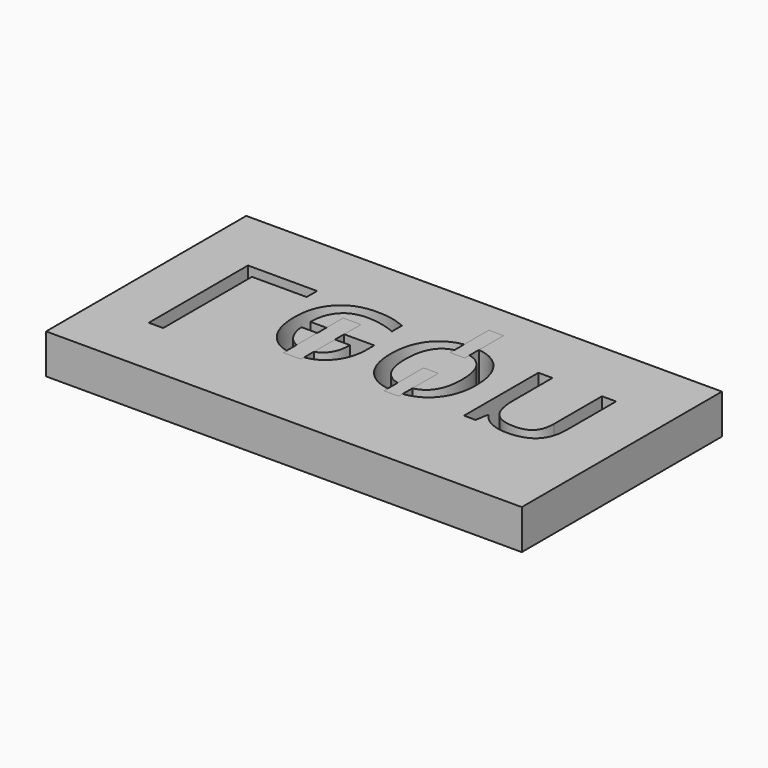
from build123d import *

# Parameters (mm, degrees)
F0_W         = 76.2
F0_H         = 40.0792241179
F1_DEPTH     = 6.35
F2_TEXT_SIZE = 27.8222769905
F3_DEPTH     = 48.006
F5_DEPTH     = 6.35
F4_W         = 2.8403475881
F4_H         = 3.3596433377


# Not quite as in the source:
# - Text() gives the source's letters only with a copy of the font that has no kerning and outlines rounded to 1/6400 em; it was checked with that copy


with BuildPart() as f1:
    # F0 (on Top) → F1 (new body)
    with BuildSketch(Plane.XY):
        Rectangle(F0_W, F0_H)
    extrude(amount=F1_DEPTH)

    # F2 (on face) → F3 (cut)
    with BuildSketch(Plane(origin=(0, 0, 0), x_dir=(1, 0, 0), z_dir=(0, 0, -1))):
        with Locations((-32.2671057508, -9.6827361845)):
            Text('Leon', F2_TEXT_SIZE, font='Open Sans', text_align=(TextAlign.LEFT, TextAlign.BOTTOM))
    extrude(amount=-F3_DEPTH, mode=Mode.SUBTRACT)


with BuildPart() as f5:
    # F4 (on face) → F5 (new body)
    with BuildSketch(Plane.XY.offset(6.35)):
        with BuildLine():
            Line((7.3115319722, 1.7436897615), (6.127636496, 1.7436897615))
            Line((6.127636496, 1.7436897615), (4.9437410198, 1.7436897615))
            Line((4.9437410198, 1.7436897615), (4.9437410198, -5.3931702091))
            add(Edge.make_bspline(
                [(4.9437410198, -5.3931702091), (5.1212427745, -5.4185774064), (5.2994799287, -5.4393437319), (5.4782769731, -5.4556621191), (5.6574797199, -5.4677304419), (5.8369560739, -5.475745273), (6.016596569, -5.4798974439), (6.2400864171, -5.4804843563), (6.2838595809, -5.4803749221), (6.3276294886, -5.4800287031), (6.3713925881, -5.4794371058), (6.4151464477, -5.4785953434), (6.4588897564, -5.4775024361), (6.6186138738, -5.4726038897), (6.7345245325, -5.4672766583), (6.8503204098, -5.4601261923), (6.965963384, -5.4510985496), (7.0814111862, -5.440139936), (7.1966174851, -5.42719747), (7.3115319723, -5.4122199485)],
                knots=[0.7306547471, 0.7306547471, 0.7306547471, 0.7306547471, 0.7306547471, 0.7306547471, 0.7306547471, 0.7306547471, 0.7570691699, 0.7570691699, 0.7570691699, 0.7570691699, 0.7570691699, 0.7570691699, 0.763502609, 0.763502609, 0.763502609, 0.763502609, 0.763502609, 0.763502609, 0.7805659698, 0.7805659698, 0.7805659698, 0.7805659698, 0.7805659698, 0.7805659698, 0.7805659698, 0.7805659698], degree=7))
            Line((7.3115319722, -5.4122199485), (7.3115319722, 1.7436897615))
        make_face()
        with BuildLine():
            add(Edge.make_bspline(
                [(4.9437410198, -5.3931702091), (5.1212427745, -5.4185774064), (5.2994799287, -5.4393437319), (5.4782769731, -5.4556621191), (5.6574797199, -5.4677304419), (5.8369560739, -5.475745273), (6.016596569, -5.4798974439), (6.2400864171, -5.4804843563), (6.2838595809, -5.4803749221), (6.3276294886, -5.4800287031), (6.3713925881, -5.4794371058), (6.4151464477, -5.4785953434), (6.4588897564, -5.4775024361), (6.6186138738, -5.4726038897), (6.7345245325, -5.4672766583), (6.8503204098, -5.4601261923), (6.965963384, -5.4510985496), (7.0814111862, -5.440139936), (7.1966174851, -5.42719747), (7.3115319723, -5.4122199485)],
                knots=[0.7306547471, 0.7306547471, 0.7306547471, 0.7306547471, 0.7306547471, 0.7306547471, 0.7306547471, 0.7306547471, 0.7570691699, 0.7570691699, 0.7570691699, 0.7570691699, 0.7570691699, 0.7570691699, 0.763502609, 0.763502609, 0.763502609, 0.763502609, 0.763502609, 0.763502609, 0.7805659698, 0.7805659698, 0.7805659698, 0.7805659698, 0.7805659698, 0.7805659698, 0.7805659698, 0.7805659698], degree=7))
            Line((4.9437410198, -5.3931702091), (4.9437410198, -6.2092860462))
            Line((4.9437410198, -6.2092860462), (7.3115319722, -6.2092860462))
            Line((7.3115319722, -6.2092860462), (7.3115319722, -5.4122199485))
        make_face()
    extrude(amount=-F5_DEPTH)


with BuildPart() as f5b:
    # F4 (on face) → F5, piece 2 (new body)
    with BuildSketch(Plane.XY.offset(6.35)):
        with BuildLine():
            Line((4.9437410198, 14.8092927411), (4.9437410198, 9.8683169196))
            add(Edge.make_bspline(
                [(7.3115319723, 9.8820572544), (7.155159451, 9.902640492), (6.9982613676, 9.9196789203), (6.8409531464, 9.9333026633), (6.6833374351, 9.9436444444), (6.5255037002, 9.950836366), (6.3675279345, 9.9550075378), (6.1535956709, 9.9567333047), (6.0977074262, 9.9568395728), (6.0418195829, 9.9565452047), (5.9859413491, 9.9558129062), (5.9300792996, 9.9546242406), (5.8742373762, 9.9529796296), (5.6928820395, 9.9462177629), (5.5674331964, 9.9392634084), (5.4421321232, 9.9299729237), (5.3170435961, 9.9182866466), (5.1922351621, 9.9041485331), (5.0677768767, 9.8875071755), (4.9437410198, 9.8683169196)],
                knots=[0.2324051313, 0.2324051313, 0.2324051313, 0.2324051313, 0.2324051313, 0.2324051313, 0.2324051313, 0.2324051313, 0.2566639921, 0.2566639921, 0.2566639921, 0.2566639921, 0.2566639921, 0.2566639921, 0.265240144, 0.265240144, 0.265240144, 0.265240144, 0.265240144, 0.265240144, 0.2845270752, 0.2845270752, 0.2845270752, 0.2845270752, 0.2845270752, 0.2845270752, 0.2845270752, 0.2845270752], degree=7))
            Line((7.3115319722, 9.8820572544), (7.3115319722, 14.8092927411))
            Line((7.3115319722, 14.8092927411), (4.9437410198, 14.8092927411))
        make_face()
        with BuildLine():
            Line((4.9437410198, 9.8683169196), (4.9437410198, 7.0456741378))
            Line((4.9437410198, 7.0456741378), (6.127636496, 7.0456741378))
            Line((6.127636496, 7.0456741378), (7.3115319722, 7.0456741378))
            Line((7.3115319722, 7.0456741378), (7.3115319722, 9.8820572544))
            add(Edge.make_bspline(
                [(7.3115319723, 9.8820572544), (7.155159451, 9.902640492), (6.9982613676, 9.9196789203), (6.8409531464, 9.9333026633), (6.6833374351, 9.9436444444), (6.5255037002, 9.950836366), (6.3675279345, 9.9550075378), (6.1535956709, 9.9567333047), (6.0977074262, 9.9568395728), (6.0418195829, 9.9565452047), (5.9859413491, 9.9558129062), (5.9300792996, 9.9546242406), (5.8742373762, 9.9529796296), (5.6928820395, 9.9462177629), (5.5674331964, 9.9392634084), (5.4421321232, 9.9299729237), (5.3170435961, 9.9182866466), (5.1922351621, 9.9041485331), (5.0677768767, 9.8875071755), (4.9437410198, 9.8683169196)],
                knots=[0.2324051313, 0.2324051313, 0.2324051313, 0.2324051313, 0.2324051313, 0.2324051313, 0.2324051313, 0.2324051313, 0.2566639921, 0.2566639921, 0.2566639921, 0.2566639921, 0.2566639921, 0.2566639921, 0.265240144, 0.265240144, 0.265240144, 0.265240144, 0.265240144, 0.265240144, 0.2845270752, 0.2845270752, 0.2845270752, 0.2845270752, 0.2845270752, 0.2845270752, 0.2845270752, 0.2845270752], degree=7))
        make_face()
    extrude(amount=-F5_DEPTH)


with BuildPart() as f5c:
    # F4 (on face) → F5, piece 3 (new body)
    with BuildSketch(Plane.XY.offset(6.35)):
        with BuildLine():
            Line((-8.500575088, 2.6445695521), (-11.340922676, 2.6445695521))
            Line((-11.340922676, 2.6445695521), (-11.340922676, -5.306372153))
            add(Edge.make_bspline(
                [(-11.340922676, -5.306372153), (-11.2953786516, -5.3168408858), (-11.2497412762, -5.3269237195), (-11.2040150626, -5.3366231645), (-11.1582044368, -5.345941875), (-11.1123137352, -5.3548826367), (-11.0663472013, -5.3634483546), (-11.020308983, -5.37164204), (-10.8215005388, -5.4053824017), (-10.6680572391, -5.4272507698), (-10.5140179464, -5.445185907), (-10.3595151105, -5.459312165), (-10.2046685578, -5.4697609958), (-10.0495851323, -5.4766677029), (-9.8943583376, -5.4801681932), (-9.6990879681, -5.4804543083), (-9.659109402, -5.4802977068), (-9.6191351942, -5.4799237764), (-9.5791678161, -5.4793302459), (-9.5392092975, -5.4785147204), (-9.4992612264, -5.4774746818), (-9.4593247488, -5.476207488), (-9.3038457034, -5.4703771896), (-9.1883997324, -5.4641191166), (-9.0731021688, -5.4558744896), (-8.9579976473, -5.4455808021), (-8.8431358023, -5.4331756131), (-8.7285711451, -5.4185974529), (-8.6143629412, -5.4017867294), (-8.500575088, -5.3826866349)],
                knots=[0.6953721092, 0.6953721092, 0.6953721092, 0.6953721092, 0.6953721092, 0.6953721092, 0.6953721092, 0.6953721092, 0.6953721092, 0.7050694305, 0.7050694305, 0.7050694305, 0.7050694305, 0.7050694305, 0.7050694305, 0.7050694305, 0.7371869593, 0.7371869593, 0.7371869593, 0.7371869593, 0.7371869593, 0.7371869593, 0.7371869593, 0.7454557222, 0.7454557222, 0.7454557222, 0.7454557222, 0.7454557222, 0.7454557222, 0.7454557222, 0.7693884814, 0.7693884814, 0.7693884814, 0.7693884814, 0.7693884814, 0.7693884814, 0.7693884814, 0.7693884814, 0.7693884814], degree=8))
            Line((-8.500575088, -5.3826866349), (-8.500575088, 2.6445695521))
        make_face()
        with Locations((-9.920748882, 4.3243912209)):
            Rectangle(F4_W, F4_H)
        with BuildLine():
            add(Edge.make_bspline(
                [(-11.340922676, -5.306372153), (-11.2953786516, -5.3168408858), (-11.2497412762, -5.3269237195), (-11.2040150626, -5.3366231645), (-11.1582044368, -5.345941875), (-11.1123137352, -5.3548826367), (-11.0663472013, -5.3634483546), (-11.020308983, -5.37164204), (-10.8215005388, -5.4053824017), (-10.6680572391, -5.4272507698), (-10.5140179464, -5.445185907), (-10.3595151105, -5.459312165), (-10.2046685578, -5.4697609958), (-10.0495851323, -5.4766677029), (-9.8943583376, -5.4801681932), (-9.6990879681, -5.4804543083), (-9.659109402, -5.4802977068), (-9.6191351942, -5.4799237764), (-9.5791678161, -5.4793302459), (-9.5392092975, -5.4785147204), (-9.4992612264, -5.4774746818), (-9.4593247488, -5.476207488), (-9.3038457034, -5.4703771896), (-9.1883997324, -5.4641191166), (-9.0731021688, -5.4558744896), (-8.9579976473, -5.4455808021), (-8.8431358023, -5.4331756131), (-8.7285711451, -5.4185974529), (-8.6143629412, -5.4017867294), (-8.500575088, -5.3826866349)],
                knots=[0.6953721092, 0.6953721092, 0.6953721092, 0.6953721092, 0.6953721092, 0.6953721092, 0.6953721092, 0.6953721092, 0.6953721092, 0.7050694305, 0.7050694305, 0.7050694305, 0.7050694305, 0.7050694305, 0.7050694305, 0.7050694305, 0.7371869593, 0.7371869593, 0.7371869593, 0.7371869593, 0.7371869593, 0.7371869593, 0.7371869593, 0.7454557222, 0.7454557222, 0.7454557222, 0.7454557222, 0.7454557222, 0.7454557222, 0.7454557222, 0.7693884814, 0.7693884814, 0.7693884814, 0.7693884814, 0.7693884814, 0.7693884814, 0.7693884814, 0.7693884814, 0.7693884814], degree=8))
            Line((-11.340922676, -5.306372153), (-11.340922676, -6.0042128898))
            Line((-11.340922676, -6.0042128898), (-8.500575088, -6.0042128898))
            Line((-8.500575088, -6.0042128898), (-8.500575088, -5.3826866349))
        make_face()
    extrude(amount=-F5_DEPTH)


solid = Compound([f1.part, f5.part, f5b.part, f5c.part])
